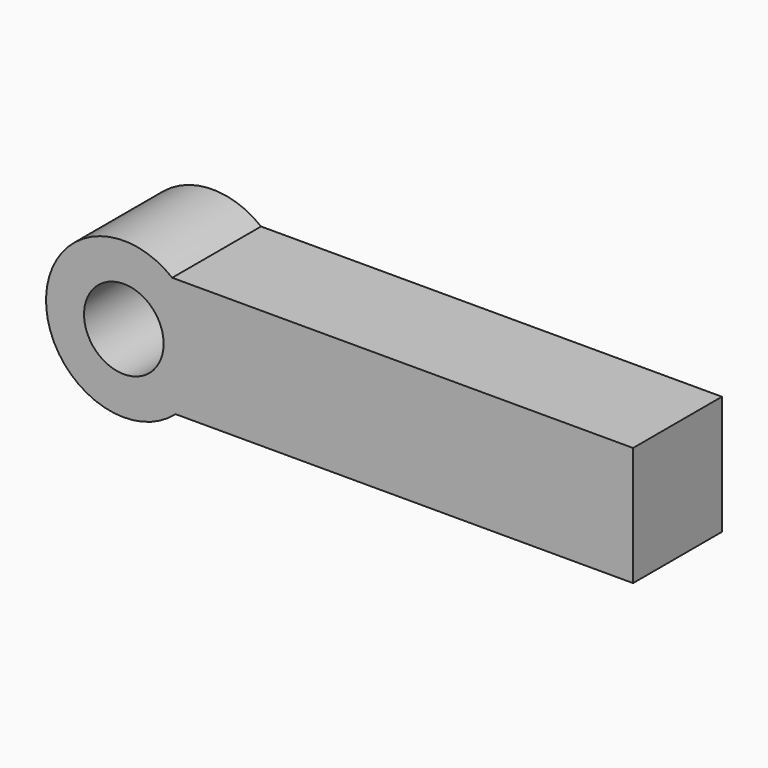
from build123d import *

# Parameters (mm, degrees)
F2_DEPTH = 30
F1_R     = 4.4049320067
F0_R     = 10.7456012025
F3_DEPTH = 30


with BuildPart() as f2:
    # F1 (on face) → F2 (new body)
    with BuildSketch(Plane.XZ):
        Polygon((-33.5293710232, 17.7000537515), (-59.1440834105, 17.7000537515), (-59.1440834105, 12.8073561937), (-42.1635434031, 12.8073561937), (-59.1440834105, -2.158543095), (-59.1440834105, -7.3390468024), (-33.2415662706, -7.3390468024), (-33.2415662706, 0), (-44.7537973523, 0), (-34.1049805284, 12.8073561937), align=None)
    extrude(amount=F2_DEPTH)


with BuildPart() as f2b:
    # F1 (on face) → F2, piece 2 (new body)
    with BuildSketch(Plane.XZ):
        with BuildLine():
            ThreePointArc((-7.7708927198, -4.3077798834), (-7.0654321008, -2.2050330991), (-6.8265853814, 0))
            ThreePointArc((-6.8265853814, 0), (-27.1834526665, 2.2050330991), (-7.7708927198, -4.3077798834))
        make_face()
        with Locations((-17.1244423836, 0)):
            Circle(F1_R, mode=Mode.SUBTRACT)
        with BuildLine():
            Line((0, -5.9000179172), (-6.8265853814, 0))
            ThreePointArc((-6.8265853814, 0), (-7.0654321008, -2.2050330991), (-7.7708927198, -4.3077798834))
            Line((-7.7708927198, -4.3077798834), (-2.5349416562, -8.8330591208))
            Line((-2.5349416562, -8.8330591208), (0, -5.9000179172))
        make_face()
    extrude(amount=F2_DEPTH)


with BuildPart() as f2c:
    # F1 (on face) → F2, piece 3 (new body)
    with BuildSketch(Plane.XZ):
        with BuildLine():
            Line((18.8512783498, 5.6122122332), (18.8512783498, 11.3683268428))
            add(Edge.make_bspline(
                [(18.8512783498, 11.3683268428), (16.934619478, 11.6522354863), (12.5645344654, 12.2995624187), (3.503068807, 6.4915593774), (1.8527053529, -3.8045495423), (8.6995157805, -9.4087929989), (15.2933857079, -8.8121851572), (18.8512783498, -8.4902700037)],
                knots=[0, 0, 0, 0, 0.1696075799, 0.3867143778, 0.5941124684, 0.7809929104, 1, 1, 1, 1], degree=3))
            Line((18.8512783498, -8.4902700037), (18.8512783498, -3.3097660635))
            add(Edge.make_bspline(
                [(18.8512783498, 5.6122122332), (17.2492587339, 5.8171733652), (14.1030304305, 6.2196993442), (10.4515493069, 3.186391092), (10.1457232334, -4.0887450053), (15.7750482612, -3.5850292061), (18.8512783498, -3.3097660635)],
                knots=[0, 0, 0, 0, 0.2323221255, 0.4562606098, 0.7028653588, 1, 1, 1, 1], degree=3))
        make_face()
    extrude(amount=F2_DEPTH)


with BuildPart() as f2d:
    # F1 (on face) → F2, piece 4 (new body)
    with BuildSketch(Plane.XZ):
        Polygon((38.4220704436, 17.1244423836), (29.7878943384, 17.1244423836), (29.7878943384, -7.6268524863), (38.4220704436, -7.6268524863), (38.4220704436, -2.4463490117), (44.4659888744, -7.3390468024), (48.7830750644, -4.8926979071), (42.7391564898, 0), (48.8952434361, 7.6045750113), (44.4659888744, 11.1901634431), (38.4220704436, 3.7241494849), align=None)
    extrude(amount=F2_DEPTH)


with BuildPart() as f2e:
    # F0 (on Front) → F2, piece 5 (new body)
    with BuildSketch(Plane.XZ):
        with BuildLine():
            ThreePointArc((-69.0952130065, 20.9325148778), (-63.2463155324, 13.6158451119), (-61.1583623106, 4.4843770224))
            ThreePointArc((-61.1583623106, 4.4843770224), (-63.0001614839, -4.1183412047), (-68.2026712705, -11.2129079295))
            Line((-68.2026712705, -11.2129079295), (55.4026070849, -11.2129079295))
            Line((55.4026070849, -11.2129079295), (55.4026070849, 20.9325148778))
            Line((55.4026070849, 20.9325148778), (-69.0952130065, 20.9325148778))
        make_face()
    extrude(amount=F2_DEPTH)


with BuildPart() as f3:
    # F0 (on Front) → F3 (new body)
    with BuildSketch(Plane.XZ):
        with BuildLine():
            ThreePointArc((-68.2026712705, -11.2129079295), (-63.0001614839, -4.1183412047), (-61.1583623106, 4.4843770224))
            ThreePointArc((-61.1583623106, 4.4843770224), (-63.2463155324, 13.6158451119), (-69.0952130065, 20.9325148778))
            ThreePointArc((-69.0952130065, 20.9325148778), (-103.1738422822, 3.901193768), (-68.2026712705, -11.2129079295))
        make_face()
        with Locations((-82.1701496464, 4.4843770224)):
            Circle(F0_R, mode=Mode.SUBTRACT)
        with BuildLine():
            ThreePointArc((-69.0952130065, 20.9325148778), (-63.2463155324, 13.6158451119), (-61.1583623106, 4.4843770224))
            ThreePointArc((-61.1583623106, 4.4843770224), (-63.0001614839, -4.1183412047), (-68.2026712705, -11.2129079295))
            Line((-68.2026712705, -11.2129079295), (55.4026070849, -11.2129079295))
            Line((55.4026070849, -11.2129079295), (55.4026070849, 20.9325148778))
            Line((55.4026070849, 20.9325148778), (-69.0952130065, 20.9325148778))
        make_face()
    extrude(amount=F3_DEPTH)


solid = Compound([f2.part, f2b.part, f2c.part, f2d.part, f2e.part, f3.part])
